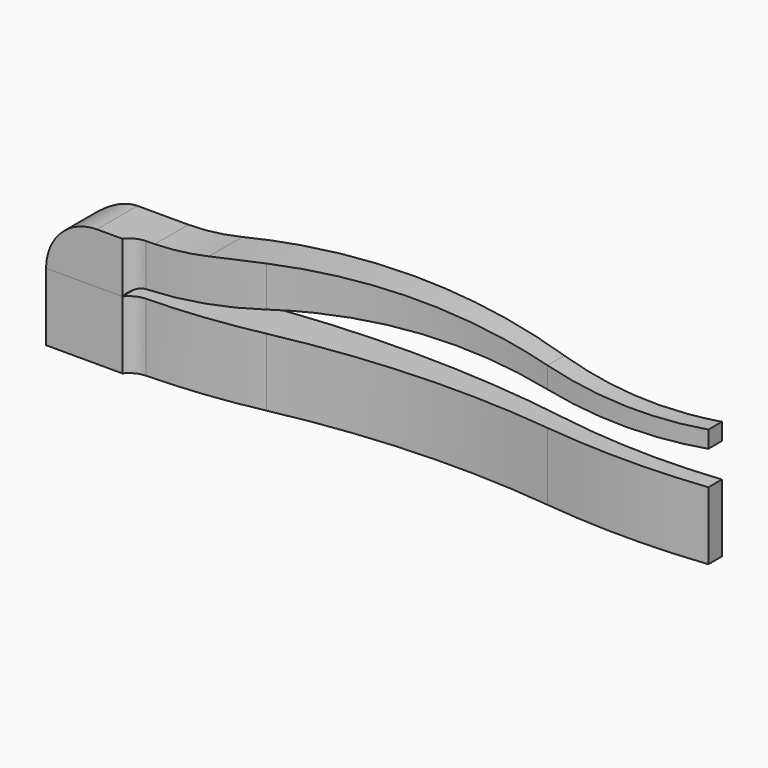
from build123d import *

# Parameters (mm, degrees)
F1_DEPTH = 40
F2_ANGLE = 90


# Not quite as in the source:
# - a feature of the source that left no trace in its solid (it failed there, or was rolled back) is left out


with BuildPart() as f1:
    # F0 (on Front) → F1 (new body, symmetric)
    with BuildSketch(Plane.XZ):
        with BuildLine():
            ThreePointArc((-315, 20), (-357.4264068712, 2.4264068712), (-375, -40))
            Line((-375, -40), (-285, -40))
            ThreePointArc((-285, -40), (-276.116980295, -32.7660394101), (-265, -30))
            ThreePointArc((-265, -30), (-199.6592526154, -25.453144), (-135, -15))
            ThreePointArc((-135, -15), (24.4030966651, 5.2339378105), (185, 0))
            ThreePointArc((185, 0), (280, -5.3255064819), (375, 0))
            Line((375, 0), (375, 20))
            ThreePointArc((375, 20), (279.8349997177, 16.2299892708), (185, 25))
            ThreePointArc((185, 25), (-5.0084565932, 39.9998115869), (-195, 24.7872720722))
            ThreePointArc((-195, 24.7872720722), (-224.9046599376, 21.198716746), (-255, 20))
            Line((-255, 20), (-315, 20))
        make_face()
    extrude(amount=F1_DEPTH, both=True)


with BuildPart() as f2_1:
    # F2: copy of F1
    add(f1.part.rotate(Axis((-330, -40, -40), (-1, 0, 0)), F2_ANGLE))


with BuildPart() as f3_1:
    # F3: copy of F2_1
    add(f2_1.part.moved(Location((0, 0, 80))))

    # F4: intersect F1
    add(f1.part, mode=Mode.INTERSECT)


solid = Compound([f2_1.part, f3_1.part])
